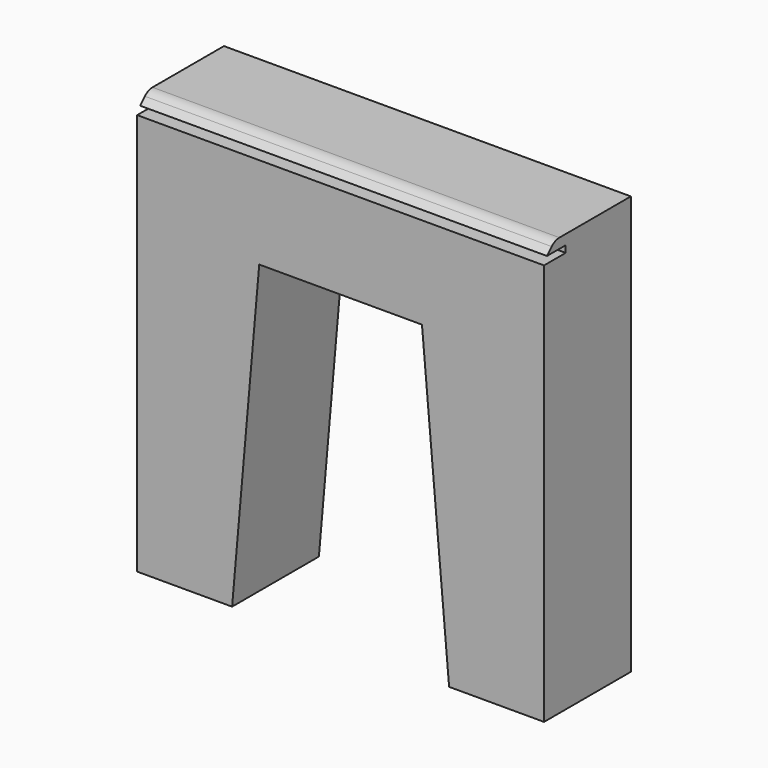
from build123d import *

# Parameters (mm, degrees)
F1_DEPTH    = 40
F2_W        = 150
F2_H        = 2.5
F3_DEPTH    = 10
F4_T1_DEPTH = 175.7168298797
F5_R        = 5


# Not quite as in the source:
# - a fillet or chamfer that OpenCascade refuses, or shapes differently, is made with other operations: its cross-section is extruded or revolved along the edge and cut away or added


with BuildPart() as f1:
    # F0 (on Front) → F1 (new body)
    with BuildSketch(Plane.XZ):
        Polygon((150, 0), (0, 0), (0, -154.3005230276), (35, -154.3005230276), (45, -40), (105, -40), (115, -154.3005230276), (150, -154.3005230276), align=None)
    extrude(amount=F1_DEPTH)

    # F2 (on face) → F3 (cut)
    with BuildSketch(Plane.XZ.offset(40)):
        with Locations((75, -4.8898250982)):
            Rectangle(F2_W, F2_H)
    extrude(amount=-F3_DEPTH, mode=Mode.SUBTRACT)

    # F4: chamfer of 5 on 1 edges, made by hand

    # F4_s2 → F4_t1 (cut)
    with BuildSketch(Plane.YZ.offset(-12.8584149398)):
        Polygon((-35, 0), (-40, -5), (-40, 0), align=None)
    extrude(amount=F4_T1_DEPTH, mode=Mode.SUBTRACT)

    # F5
    f5_edges = [f1.edges().sort_by_distance(p)[0] for p in [
        (75, -35, 0),
    ]]
    fillet(f5_edges, radius=F5_R)


solid = f1.part
